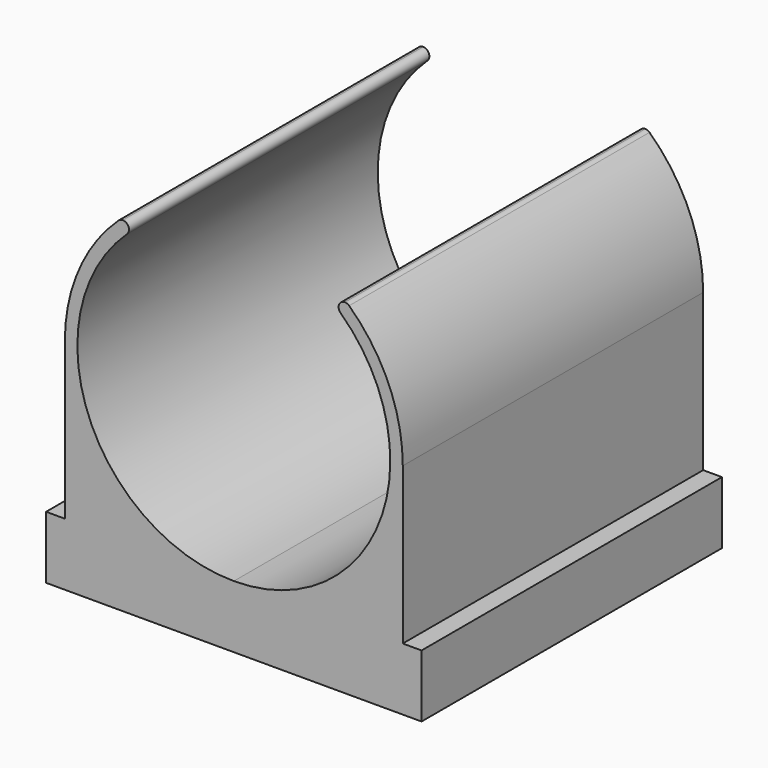
from build123d import *

# Parameters (mm, degrees)
F1_W     = 30
F1_H     = 30
F2_DEPTH = 5
F3_DEPTH = 15
F4_R     = 0.49999


# Not quite as in the source:
# - a fillet or chamfer is up to 0.001 mm smaller than in the source, because OpenCascade refuses the exact size


with BuildPart() as f2:
    # F1 (on Top) → F2 (new body)
    with BuildSketch(Plane.XY):
        Rectangle(F1_W, F1_H)
    extrude(amount=-F2_DEPTH)

    # F0 (on Front) → F3 (join, symmetric)
    with BuildSketch(Plane.XZ):
        with BuildLine():
            ThreePointArc((0, 0), (-11.8585412256, 8.5471529248), (-7.5, 22.5))
            Line((-7.5, 22.5), (-9.0691785736, 22.5))
            ThreePointArc((-9.0691785736, 22.5), (-12.3426883365, 17.9688247941), (-13.5, 12.5))
            Line((-13.5, 12.5), (-13.5, 0))
            Line((-13.5, 0), (0, 0))
        make_face()
        with BuildLine():
            ThreePointArc((7.5, 22.5), (11.8585412256, 8.5471529248), (0, 0))
            Line((0, 0), (13.5, 0))
            Line((13.5, 0), (13.5, 12.5))
            ThreePointArc((13.5, 12.5), (12.3426883365, 17.9688247941), (9.0691785736, 22.5))
            Line((9.0691785736, 22.5), (7.5, 22.5))
        make_face()
    extrude(amount=F3_DEPTH, both=True)

    # F4 (radius 0.5 in the source; OpenCascade refuses exactly that, so slightly less here)
    f4_edges = [f2.edges().sort_by_distance(p)[0] for p in [
        (-7.5, 0, 22.5),
        (9.069179, 0, 22.5),
        (-9.069179, 0, 22.5),
        (7.5, 0, 22.5),
    ]]
    fillet(f4_edges, radius=F4_R)


solid = f2.part
